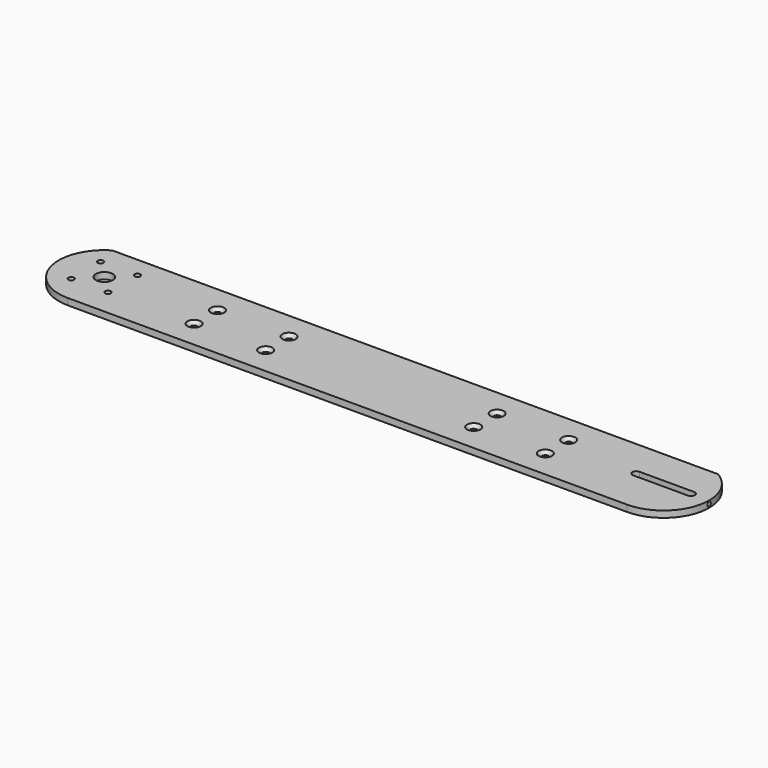
from build123d import *

# Parameters (mm, degrees)
F0_R     = 3.4
F0_R_2   = 5.25
F0_R_3   = 13
F1_DEPTH = 10
F3_D     = 8.8
F5_R     = 3.25
F6_DEPTH = 43.0009999364
F7_SIZE  = 5
F8_SIZE  = 5
F9_SIZE  = 4.99999


# Not quite as in the source:
# - a fillet or chamfer is up to 0.001 mm smaller than in the source, because OpenCascade refuses the exact size
# - ends of sketch curves that miss each other by under 0.0002 mm in the source are joined


with BuildPart() as f1:
    # F0 (on Top) → F1 (new body)
    with BuildSketch(Plane.XY):
        with BuildLine():
            Line((466.055512, 65), (-466.055513, 65))
            ThreePointArc((-466.055513, 65), (-497.4536877881, -13.7082870352), (-430, -65))
            Line((-430, -65), (430, -65))
            ThreePointArc((430, -65), (497.4536879026, -13.7082866222), (466.055512, 65))
        make_face()
        with Locations((-458.285, -23.285)):
            Circle(F0_R, mode=Mode.SUBTRACT)
        with Locations((-401.715, -23.285)):
            Circle(F0_R, mode=Mode.SUBTRACT)
        with Locations((-270, -22.5)):
            Circle(F0_R_2, mode=Mode.SUBTRACT)
        with Locations((-160, -22.5)):
            Circle(F0_R_2, mode=Mode.SUBTRACT)
        with Locations((160, -22.5)):
            Circle(F0_R_2, mode=Mode.SUBTRACT)
        with Locations((270, -22.5)):
            Circle(F0_R_2, mode=Mode.SUBTRACT)
        with Locations((-430, 5)):
            Circle(F0_R_3, mode=Mode.SUBTRACT)
        with Locations((-270, 22.5)):
            Circle(F0_R_2, mode=Mode.SUBTRACT)
        with Locations((-160, 22.5)):
            Circle(F0_R_2, mode=Mode.SUBTRACT)
        with Locations((-458.285, 33.285)):
            Circle(F0_R, mode=Mode.SUBTRACT)
        with Locations((-401.715, 33.285)):
            Circle(F0_R, mode=Mode.SUBTRACT)
        with Locations((160, 22.5)):
            Circle(F0_R_2, mode=Mode.SUBTRACT)
        with BuildLine():
            ThreePointArc((471.997057, 10.999994999), (477.9971689997, 5.000051), (471.997169, -1.000005))
            Line((471.997169, -1.000005), (387.989411, -1))
            ThreePointArc((387.989411, -1), (381.9976061696, 5.0724232034), (388.1342589922, 10.9984286567))
            Line((388.1342589922, 10.9984286567), (471.997057, 10.999994999))
        make_face(mode=Mode.SUBTRACT)
        with Locations((270, 22.5)):
            Circle(F0_R_2, mode=Mode.SUBTRACT)
    extrude(amount=F1_DEPTH)

    # F3 (through all)
    with Locations(Plane.XY.offset(10)):
        with Locations((-458.285, -23.285), (-401.715, -23.285), (-401.715, 33.285), (-458.285, 33.285)):
            Hole(F3_D / 2)

    # F5 (on offset) → F6 (cut, through all)
    with BuildSketch(Plane.YZ.offset(457)):
        with Locations((5, 5)):
            Circle(F5_R)
    extrude(amount=F6_DEPTH, mode=Mode.SUBTRACT)

    # F7
    f7_edges = [f1.edges().sort_by_distance(p)[0] for p in [
        (-275.25, -22.5, 10),
        (-275.25, 22.5, 10),
        (-165.25, -22.5, 10),
        (-165.25, 22.5, 10),
    ]]
    chamfer(f7_edges, length=F7_SIZE)

    # F8
    f8_edges = [f1.edges().sort_by_distance(p)[0] for p in [
        (264.75, 22.5, 10),
        (264.75, -22.5, 10),
        (154.75, -22.5, 10),
        (154.75, 22.5, 10),
    ]]
    chamfer(f8_edges, length=F8_SIZE)

    # F9 (size 5 in the source; OpenCascade refuses exactly that, so slightly less here)
    f9_edges = [f1.edges().sort_by_distance(p)[0] for p in [
        (264.75, -22.5, 0),
        (264.75, 22.5, 0),
        (154.75, 22.5, 0),
        (154.75, -22.5, 0),
        (-165.25, 22.5, 0),
        (-165.25, -22.5, 0),
        (-275.25, 22.5, 0),
        (-275.25, -22.5, 0),
    ]]
    chamfer(f9_edges, length=F9_SIZE)


solid = f1.part
